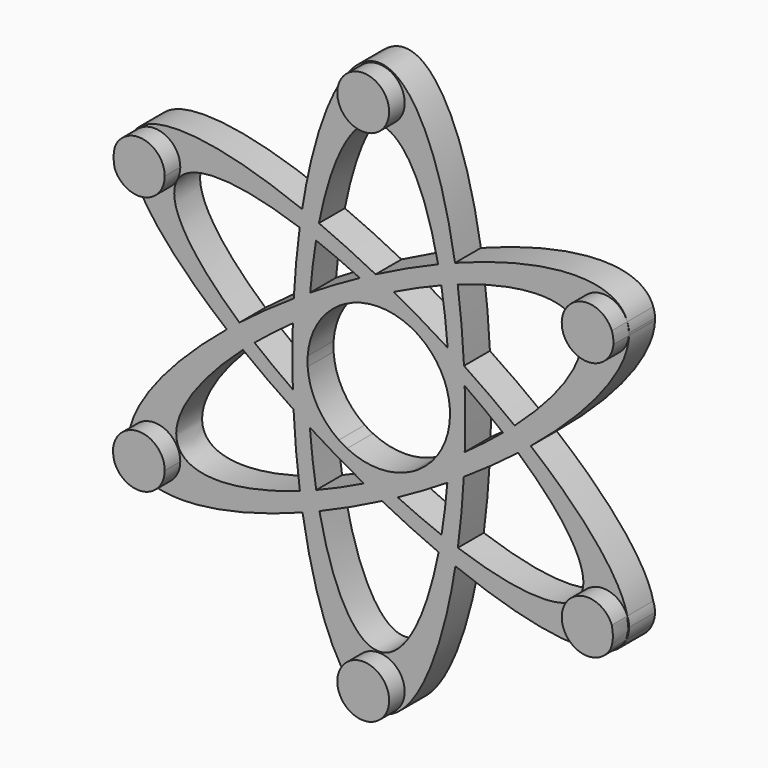
from build123d import *

# Parameters (mm, degrees)
F0_R     = 4
F1_DEPTH = 8
F2_DEPTH = 5


with BuildPart() as f1:
    # F0 (on Front) → F1 (new body)
    with BuildSketch(Plane.XZ):
        with Locations((0, 40)):
            Circle(F0_R)
    extrude(amount=F1_DEPTH)


with BuildPart() as f1b:
    # F0 (on Front) → F1, piece 2 (new body)
    with BuildSketch(Plane.XZ):
        with Locations((0, -40)):
            Circle(F0_R)
    extrude(amount=F1_DEPTH)


with BuildPart() as f1c:
    # F0 (on Front) → F1, piece 3 (new body)
    with BuildSketch(Plane.XZ):
        with BuildLine():
            add(Edge.make_bspline(
                [(38.6271723405, 19.6674961115), (38.6460169038, 20.6376327061), (38.3690323303, 21.4497914918)],
                knots=[2.9551502566, 2.9551502566, 2.9551502566, 3.0789616265, 3.0789616265, 3.0789616265], degree=2, weights=[1, 0.998084455, 1]))
            ThreePointArc((38.3690323303, 21.4497914918), (30.6823221702, 19.4266397613), (38.6271723405, 19.6674961115))
        make_face()
    extrude(amount=F1_DEPTH)


with BuildPart() as f1d:
    # F0 (on Front) → F1, piece 4 (new body)
    with BuildSketch(Plane.XZ):
        with BuildLine():
            add(Edge.make_bspline(
                [(38.1831586596, -21.8582858906), (38.7767020629, -20.4672732588), (38.3678501734, -18.5471723529)],
                knots=[3.1799341158, 3.1799341158, 3.1799341158, 3.4078051361, 3.4078051361, 3.4078051361], degree=2, weights=[1, 0.9935163681, 1]))
            ThreePointArc((38.3678501734, -18.5471723529), (30.6472243235, -19.7772291859), (38.1831586596, -21.8582858906))
        make_face()
    extrude(amount=F1_DEPTH)


with BuildPart() as f1e:
    # F0 (on Front) → F1, piece 5 (new body)
    with BuildSketch(Plane.XZ):
        with BuildLine():
            ThreePointArc((-30.6410161514, 20), (-33.684086173, 23.8838492526), (-38.1831586596, 21.8582858906))
            add(Edge.make_bspline(
                [(-38.1831586596, 21.8582858906), (-38.7767020629, 20.4672732588), (-38.3678501734, 18.5471723529)],
                knots=[0.0383414622, 0.0383414622, 0.0383414622, 0.2662124825, 0.2662124825, 0.2662124825], degree=2, weights=[1, 0.9935163681, 1]))
            ThreePointArc((-38.3678501734, 18.5471723529), (-33.9018734345, 16.068884631), (-30.6410161514, 20))
        make_face()
    extrude(amount=F1_DEPTH)


with BuildPart() as f1f:
    # F0 (on Front) → F1, piece 6 (new body)
    with BuildSketch(Plane.XZ):
        with BuildLine():
            ThreePointArc((-30.6410161514, -20), (-34.4746201727, -16.0034624513), (-38.6271723405, -19.6674961115))
            add(Edge.make_bspline(
                [(-38.6271723405, -19.6674961115), (-38.6460169038, -20.6376327061), (-38.3690323303, -21.4497914918)],
                knots=[6.0967429102, 6.0967429102, 6.0967429102, 6.2205542801, 6.2205542801, 6.2205542801], degree=2, weights=[1, 0.998084455, 1]))
            ThreePointArc((-38.3690323303, -21.4497914918), (-33.9034745307, -23.9314160754), (-30.6410161514, -20))
        make_face()
    extrude(amount=F1_DEPTH)


with BuildPart() as f2:
    # F0 (on Front) → F2 (new body)
    with BuildSketch(Plane.XZ):
        with BuildLine():
            ThreePointArc((38.6271723405, 19.6674961115), (38.6375537001, 19.8336040213), (38.6410161514, 20))
            ThreePointArc((38.6410161514, 20), (38.5724322268, 20.7375416206), (38.3690323303, 21.4497914918))
            add(Edge.make_bspline(
                [(38.6271723405, 19.6674961115), (38.6460169038, 20.6376327061), (38.3690323303, 21.4497914918)],
                knots=[2.9551502566, 2.9551502566, 2.9551502566, 3.0789616265, 3.0789616265, 3.0789616265], degree=2, weights=[1, 0.998084455, 1]))
        make_face()
        with BuildLine():
            add(Edge.make_bspline(
                [(38.6271723405, 19.6674961115), (38.6460169038, 20.6376327061), (38.3690323303, 21.4497914918)],
                knots=[2.9551502566, 2.9551502566, 2.9551502566, 3.0789616265, 3.0789616265, 3.0789616265], degree=2, weights=[1, 0.998084455, 1]))
            ThreePointArc((38.3690323303, 21.4497914918), (30.6823221702, 19.4266397613), (38.6271723405, 19.6674961115))
        make_face()
        with BuildLine():
            ThreePointArc((38.6271723405, 19.6674961115), (30.6823221702, 19.4266397613), (38.3690323303, 21.4497914918))
            add(Edge.make_bspline(
                [(38.3690323303, 21.4497914918), (35.4881888834, 29.8968406764), (11.768870068, 20.7886243591)],
                knots=[3.0789616265, 3.0789616265, 3.0789616265, 4.224226026, 4.224226026, 4.224226026], degree=2, weights=[1, 0.8404776409, 1]))
            add(Edge.make_bspline(
                [(11.768870068, 20.7886243591), (-0.1383581355, 94.7656935014), (-11.8290209253, 20.4105265383)],
                knots=[5.2022540895, 5.2022540895, 5.2022540895, 7.3737896961, 7.3737896961, 7.3737896961], degree=2, weights=[1, 0.4662335933, 1]))
            add(Edge.make_bspline(
                [(-11.8290209253, 20.4105265383), (-34.91761313, 29.5113320816), (-38.1831586596, 21.8582858906)],
                knots=[5.1977622276, 5.1977622276, 5.1977622276, 6.3215267693, 6.3215267693, 6.3215267693], degree=2, weights=[1, 0.8462537744, 1]))
            ThreePointArc((-38.1831586596, 21.8582858906), (-33.684086173, 23.8838492526), (-30.6410161514, 20))
            ThreePointArc((-30.6410161514, 20), (-33.9018734345, 16.068884631), (-38.3678501734, 18.5471723529))
            add(Edge.make_bspline(
                [(-38.3678501734, 18.5471723529), (-36.8074034343, 11.2188090154), (-23.4546094015, 0.2961662725)],
                knots=[0.2662124825, 0.2662124825, 0.2662124825, 1.0897639985, 1.0897639985, 1.0897639985], degree=2, weights=[1, 0.9164115435, 1]))
            add(Edge.make_bspline(
                [(-23.4546094015, 0.2961662725), (-38.4783576877, -12.0063718778), (-38.6271723405, -19.6674961115)],
                knots=[5.1863313593, 5.1863313593, 5.1863313593, 6.0967429102, 6.0967429102, 6.0967429102], degree=2, weights=[1, 0.8981705786, 1]))
            ThreePointArc((-38.6271723405, -19.6674961115), (-34.4746201727, -16.0034624513), (-30.6410161514, -20))
            ThreePointArc((-30.6410161514, -20), (-33.9034745307, -23.9314160754), (-38.3690323303, -21.4497914918))
            add(Edge.make_bspline(
                [(-38.3690323303, -21.4497914918), (-35.4881888834, -29.8968406764), (-11.768870068, -20.7886243591)],
                knots=[6.2205542801, 6.2205542801, 6.2205542801, 7.3658186796, 7.3658186796, 7.3658186796], degree=2, weights=[1, 0.8404776409, 1]))
            add(Edge.make_bspline(
                [(-11.768870068, -20.7886243591), (0.1383581355, -94.7656935014), (11.8290209253, -20.4105265383)],
                knots=[2.060661436, 2.060661436, 2.060661436, 4.2321970425, 4.2321970425, 4.2321970425], degree=2, weights=[1, 0.4662335933, 1]))
            add(Edge.make_bspline(
                [(11.8290209253, -20.4105265383), (34.91761313, -29.5113320816), (38.1831586596, -21.8582858906)],
                knots=[2.056169574, 2.056169574, 2.056169574, 3.1799341158, 3.1799341158, 3.1799341158], degree=2, weights=[1, 0.8462537744, 1]))
            ThreePointArc((38.1831586596, -21.8582858906), (30.6472243235, -19.7772291859), (38.3678501734, -18.5471723529))
            add(Edge.make_bspline(
                [(38.3678501734, -18.5471723529), (36.8074034343, -11.2188090154), (23.4546094015, -0.2961662725)],
                knots=[3.4078051361, 3.4078051361, 3.4078051361, 4.231356652, 4.231356652, 4.231356652], degree=2, weights=[1, 0.9164115435, 1]))
            add(Edge.make_bspline(
                [(23.4546094015, -0.2961662725), (38.4783576877, 12.0063718778), (38.6271723405, 19.6674961115)],
                knots=[2.0447387057, 2.0447387057, 2.0447387057, 2.9551502566, 2.9551502566, 2.9551502566], degree=2, weights=[1, 0.8981705786, 1]))
        make_face()
        with BuildLine():
            add(Edge.make_bspline(
                [(-20.9775166101, -1.6715988722), (-57.3346911932, -34.0027613149), (-12.1812992651, -17.9934813476)],
                knots=[5.2662721481, 5.2662721481, 5.2662721481, 7.272346213, 7.272346213, 7.272346213], degree=2, weights=[1, 0.5377442434, 1]))
            add(Edge.make_bspline(
                [(-20.9775166101, -1.6715988722), (-17.2892670675, -4.5190906219), (-13.156595617, -7.250418808)],
                knots=[1.1684900965, 1.1684900965, 1.1684900965, 1.3957166856, 1.3957166856, 1.3957166856], degree=2, weights=[1, 0.993552949, 1]))
            add(Edge.make_bspline(
                [(-13.156595617, -7.250418808), (-12.8764761834, -12.8287089611), (-12.1812992651, -17.9934813476)],
                knots=[1.73563988, 1.73563988, 1.73563988, 1.9902315228, 1.9902315228, 1.9902315228], degree=2, weights=[1, 0.9919088217, 1]))
        make_face(mode=Mode.SUBTRACT)
        with BuildLine():
            add(Edge.make_bspline(
                [(-10.6355871975, -8.8788558816), (-10.3001887138, -13.1602609633), (-9.6562230523, -17.0474184543)],
                knots=[1.8211625389, 1.8211625389, 1.8211625389, 2.0665528838, 2.0665528838, 2.0665528838], degree=2, weights=[1, 0.9924823853, 1]))
            add(Edge.make_bspline(
                [(-10.6355871975, -8.8788558816), (-6.5457802924, -11.4608048965), (-2.2982627366, -13.7666231954)],
                knots=[1.4645175631, 1.4645175631, 1.4645175631, 1.6844760114, 1.6844760114, 1.6844760114], degree=2, weights=[1, 0.9939583785, 1]))
            add(Edge.make_bspline(
                [(-9.6562230523, -17.0474184543), (-6.06442069, -15.6317314707), (-2.2982627366, -13.7666231954)],
                knots=[1.0753748884, 1.0753748884, 1.0753748884, 1.3157471354, 1.3157471354, 1.3157471354], degree=2, weights=[1, 0.9927863374, 1]))
        make_face(mode=Mode.SUBTRACT)
        with BuildLine():
            add(Edge.make_bspline(
                [(-13.2699308243, 4.4384553681), (-16.4241224972, 2.1873919184), (-19.1756694614, -0.1172964225)],
                knots=[4.9691723309, 4.9691723309, 4.9691723309, 5.191056423, 5.191056423, 5.191056423], degree=2, weights=[1, 0.9938522407, 1]))
            add(Edge.make_bspline(
                [(-13.2699308243, 4.4384553681), (-13.4070301609, -0.0598567192), (-13.2662713173, -4.5569282873)],
                knots=[1.4701714839, 1.4701714839, 1.4701714839, 1.674116558, 1.674116558, 1.674116558], degree=2, weights=[1, 0.9948053046, 1]))
            add(Edge.make_bspline(
                [(-19.1756694614, -0.1172964225), (-16.4170834766, -2.3653682673), (-13.2662713173, -4.5569282873)],
                knots=[1.094094817, 1.094094817, 1.094094817, 1.3131248908, 1.3131248908, 1.3131248908], degree=2, weights=[1, 0.9940092195, 1]))
        make_face(mode=Mode.SUBTRACT)
        with Locations((0, -40)):
            Circle(F0_R, mode=Mode.SUBTRACT)
        with BuildLine():
            add(Edge.make_bspline(
                [(-9.1608560146, -19.7471255553), (-4.4037766582, -17.7758354546), (0.4925988488, -15.2422767275)],
                knots=[1.1527895646, 1.1527895646, 1.1527895646, 1.40497696, 1.40497696, 1.40497696], degree=2, weights=[1, 0.9920607174, 1]))
            add(Edge.make_bspline(
                [(0.4925988488, -15.2422767275), (4.9307327719, -17.5263667759), (9.2397434736, -19.3514863138)],
                knots=[1.7569380094, 1.7569380094, 1.7569380094, 1.9862959493, 1.9862959493, 1.9862959493], degree=2, weights=[1, 0.9934315703, 1]))
            add(Edge.make_bspline(
                [(-9.1608560146, -19.7471255553), (0.1325416539, -65.6909824303), (9.2397434736, -19.3514863138)],
                knots=[2.1543953797, 2.1543953797, 2.1543953797, 4.1419628072, 4.1419628072, 4.1419628072], degree=2, weights=[1, 0.5455226575, 1]))
        make_face(mode=Mode.SUBTRACT)
        with BuildLine():
            add(Edge.make_bspline(
                [(2.9247407794, -13.9530221579), (6.381572516, -15.5960962195), (9.6859688453, -16.866629301)],
                knots=[1.8394563331, 1.8394563331, 1.8394563331, 2.0584655411, 2.0584655411, 2.0584655411], degree=2, weights=[1, 0.9940103597, 1]))
            add(Edge.make_bspline(
                [(2.9247407794, -13.9530221579), (6.8250937635, -11.8359876839), (10.5868988303, -9.4786852371)],
                knots=[1.4680117284, 1.4680117284, 1.4680117284, 1.6698474867, 1.6698474867, 1.6698474867], degree=2, weights=[1, 0.9949121111, 1]))
            add(Edge.make_bspline(
                [(9.6859688453, -16.866629301), (10.2627564961, -13.3368180686), (10.5868988303, -9.4786852371)],
                knots=[4.2223588686, 4.2223588686, 4.2223588686, 4.4447070614, 4.4447070614, 4.4447070614], degree=2, weights=[1, 0.9938265226, 1]))
        make_face(mode=Mode.SUBTRACT)
        with BuildLine():
            add(Edge.make_bspline(
                [(12.2086468073, -17.7889135993), (12.8445989111, -12.9990853571), (13.1252234213, -7.8496558732)],
                knots=[4.2980174693, 4.2980174693, 4.2980174693, 4.533780381, 4.533780381, 4.533780381], degree=2, weights=[1, 0.9930600233, 1]))
            add(Edge.make_bspline(
                [(13.1252234213, -7.8496558732), (17.5751199012, -4.9249756496), (21.5054671299, -1.8547051014)],
                knots=[1.7389094291, 1.7389094291, 1.7389094291, 1.9826652124, 1.9826652124, 1.9826652124], degree=2, weights=[1, 0.9925820789, 1]))
            add(Edge.make_bspline(
                [(12.2086468073, -17.7889135993), (57.3364841528, -33.4072559177), (21.5054671299, -1.8547051014)],
                knots=[2.1436727474, 2.1436727474, 2.1436727474, 4.139111996, 4.139111996, 4.139111996], degree=2, weights=[1, 0.5422197693, 1]))
        make_face(mode=Mode.SUBTRACT)
        with BuildLine():
            add(Edge.make_bspline(
                [(-12.2086468073, 17.7889135993), (-12.8445989111, 12.9990853571), (-13.1252234213, 7.8496558732)],
                knots=[1.1564248157, 1.1564248157, 1.1564248157, 1.3921877274, 1.3921877274, 1.3921877274], degree=2, weights=[1, 0.9930600233, 1]))
            add(Edge.make_bspline(
                [(-13.1252234213, 7.8496558732), (-17.5751199012, 4.9249756496), (-21.5054671299, 1.8547051014)],
                knots=[4.8805020827, 4.8805020827, 4.8805020827, 5.1242578659, 5.1242578659, 5.1242578659], degree=2, weights=[1, 0.9925820789, 1]))
            add(Edge.make_bspline(
                [(-12.2086468073, 17.7889135993), (-57.3364841528, 33.4072559177), (-21.5054671299, 1.8547051014)],
                knots=[5.2852654009, 5.2852654009, 5.2852654009, 7.2807046496, 7.2807046496, 7.2807046496], degree=2, weights=[1, 0.5422197693, 1]))
        make_face(mode=Mode.SUBTRACT)
        with BuildLine():
            add(Edge.make_bspline(
                [(-2.9247407794, 13.9530221579), (-6.381572516, 15.5960962195), (-9.6859688453, 16.866629301)],
                knots=[4.9810489867, 4.9810489867, 4.9810489867, 5.2000581947, 5.2000581947, 5.2000581947], degree=2, weights=[1, 0.9940103597, 1]))
            add(Edge.make_bspline(
                [(-2.9247407794, 13.9530221579), (-6.8250937635, 11.8359876839), (-10.5868988303, 9.4786852371)],
                knots=[4.6096043819, 4.6096043819, 4.6096043819, 4.8114401403, 4.8114401403, 4.8114401403], degree=2, weights=[1, 0.9949121111, 1]))
            add(Edge.make_bspline(
                [(-9.6859688453, 16.866629301), (-10.2627564961, 13.3368180686), (-10.5868988303, 9.4786852371)],
                knots=[1.080766215, 1.080766215, 1.080766215, 1.3031144078, 1.3031144078, 1.3031144078], degree=2, weights=[1, 0.9938265226, 1]))
        make_face(mode=Mode.SUBTRACT)
        with BuildLine():
            add(Edge.make_bspline(
                [(9.1608560146, 19.7471255553), (4.4037766582, 17.7758354546), (-0.4925988488, 15.2422767275)],
                knots=[4.2943822182, 4.2943822182, 4.2943822182, 4.5465696136, 4.5465696136, 4.5465696136], degree=2, weights=[1, 0.9920607174, 1]))
            add(Edge.make_bspline(
                [(-0.4925988488, 15.2422767275), (-4.9307327719, 17.5263667759), (-9.2397434736, 19.3514863138)],
                knots=[4.898530663, 4.898530663, 4.898530663, 5.1278886029, 5.1278886029, 5.1278886029], degree=2, weights=[1, 0.9934315703, 1]))
            add(Edge.make_bspline(
                [(9.1608560146, 19.7471255553), (-0.1325416539, 65.6909824303), (-9.2397434736, 19.3514863138)],
                knots=[5.2959880333, 5.2959880333, 5.2959880333, 7.2835554608, 7.2835554608, 7.2835554608], degree=2, weights=[1, 0.5455226575, 1]))
        make_face(mode=Mode.SUBTRACT)
        with BuildLine():
            ThreePointArc((10.9755620079, 0.7328291827), (10.9938888044, 0.366618271), (11, 0))
            ThreePointArc((11, 0), (10.9938888044, -0.366618271), (10.9755620079, -0.7328291827))
            ThreePointArc((10.9755620079, -0.7328291827), (9.5348282556, -5.4851663728), (6.1508474506, -9.1195984363))
            ThreePointArc((6.1508474506, -9.1195984363), (5.6512634903, -9.4373312416), (5.1353077604, -9.7277239993))
            ThreePointArc((5.1353077604, -9.7277239993), (0.1365678891, -10.9991522042), (-4.8921987801, -9.8522277225))
            ThreePointArc((-4.8921987801, -9.8522277225), (-5.5371729973, -9.5047206797), (-6.1575844575, -9.1150509405))
            ThreePointArc((-6.1575844575, -9.1150509405), (-9.5368541643, -5.4816432435), (-10.9755620079, -0.7328291827))
            ThreePointArc((-10.9755620079, -0.7328291827), (-11, 0), (-10.9755620079, 0.7328291827))
            ThreePointArc((-10.9755620079, 0.7328291827), (-9.5348282556, 5.4851663728), (-6.1508474506, 9.1195984363))
            ThreePointArc((-6.1508474506, 9.1195984363), (-5.6512634903, 9.4373312416), (-5.1353077604, 9.7277239993))
            ThreePointArc((-5.1353077604, 9.7277239993), (-0.1365678891, 10.9991522042), (4.8921987801, 9.8522277225))
            ThreePointArc((4.8921987801, 9.8522277225), (5.5371729973, 9.5047206797), (6.1575844575, 9.1150509405))
            ThreePointArc((6.1575844575, 9.1150509405), (9.5368541643, 5.4816432435), (10.9755620079, 0.7328291827))
        make_face(mode=Mode.SUBTRACT)
        with BuildLine():
            add(Edge.make_bspline(
                [(13.2699308243, -4.4384553681), (16.4241224972, -2.1873919184), (19.1756694614, 0.1172964225)],
                knots=[1.8275796773, 1.8275796773, 1.8275796773, 2.0494637694, 2.0494637694, 2.0494637694], degree=2, weights=[1, 0.9938522407, 1]))
            add(Edge.make_bspline(
                [(13.2699308243, -4.4384553681), (13.4070301609, 0.0598567192), (13.2662713173, 4.5569282873)],
                knots=[4.6117641375, 4.6117641375, 4.6117641375, 4.8157092116, 4.8157092116, 4.8157092116], degree=2, weights=[1, 0.9948053046, 1]))
            add(Edge.make_bspline(
                [(19.1756694614, 0.1172964225), (16.4170834766, 2.3653682673), (13.2662713173, 4.5569282873)],
                knots=[4.2356874706, 4.2356874706, 4.2356874706, 4.4547175444, 4.4547175444, 4.4547175444], degree=2, weights=[1, 0.9940092195, 1]))
        make_face(mode=Mode.SUBTRACT)
        with BuildLine():
            add(Edge.make_bspline(
                [(10.6355871975, 8.8788558816), (10.3001887138, 13.1602609633), (9.6562230523, 17.0474184543)],
                knots=[4.9627551925, 4.9627551925, 4.9627551925, 5.2081455374, 5.2081455374, 5.2081455374], degree=2, weights=[1, 0.9924823853, 1]))
            add(Edge.make_bspline(
                [(10.6355871975, 8.8788558816), (6.5457802924, 11.4608048965), (2.2982627366, 13.7666231954)],
                knots=[4.6061102167, 4.6061102167, 4.6061102167, 4.826068665, 4.826068665, 4.826068665], degree=2, weights=[1, 0.9939583785, 1]))
            add(Edge.make_bspline(
                [(9.6562230523, 17.0474184543), (6.06442069, 15.6317314707), (2.2982627366, 13.7666231954)],
                knots=[4.216967542, 4.216967542, 4.216967542, 4.457339789, 4.457339789, 4.457339789], degree=2, weights=[1, 0.9927863374, 1]))
        make_face(mode=Mode.SUBTRACT)
        with BuildLine():
            add(Edge.make_bspline(
                [(20.9775166101, 1.6715988722), (17.2892670675, 4.5190906219), (13.156595617, 7.250418808)],
                knots=[4.3100827501, 4.3100827501, 4.3100827501, 4.5373093392, 4.5373093392, 4.5373093392], degree=2, weights=[1, 0.993552949, 1]))
            add(Edge.make_bspline(
                [(13.156595617, 7.250418808), (12.8764761834, 12.8287089611), (12.1812992651, 17.9934813476)],
                knots=[4.8772325336, 4.8772325336, 4.8772325336, 5.1318241764, 5.1318241764, 5.1318241764], degree=2, weights=[1, 0.9919088217, 1]))
            add(Edge.make_bspline(
                [(20.9775166101, 1.6715988722), (57.3346911932, 34.0027613149), (12.1812992651, 17.9934813476)],
                knots=[2.1246794946, 2.1246794946, 2.1246794946, 4.1307535594, 4.1307535594, 4.1307535594], degree=2, weights=[1, 0.5377442434, 1]))
        make_face(mode=Mode.SUBTRACT)
        with Locations((0, 40)):
            Circle(F0_R, mode=Mode.SUBTRACT)
        with BuildLine():
            add(Edge.make_bspline(
                [(38.1831586596, -21.8582858906), (38.7767020629, -20.4672732588), (38.3678501734, -18.5471723529)],
                knots=[3.1799341158, 3.1799341158, 3.1799341158, 3.4078051361, 3.4078051361, 3.4078051361], degree=2, weights=[1, 0.9935163681, 1]))
            ThreePointArc((38.3678501734, -18.5471723529), (30.6472243235, -19.7772291859), (38.1831586596, -21.8582858906))
        make_face()
        with BuildLine():
            ThreePointArc((38.6410161514, -20), (38.5721315203, -19.2608572831), (38.3678501734, -18.5471723529))
            add(Edge.make_bspline(
                [(38.1831586596, -21.8582858906), (38.7767020629, -20.4672732588), (38.3678501734, -18.5471723529)],
                knots=[3.1799341158, 3.1799341158, 3.1799341158, 3.4078051361, 3.4078051361, 3.4078051361], degree=2, weights=[1, 0.9935163681, 1]))
            ThreePointArc((38.1831586596, -21.8582858906), (38.5248654039, -20.9569299783), (38.6410161514, -20))
        make_face()
        with BuildLine():
            add(Edge.make_bspline(
                [(-38.1831586596, 21.8582858906), (-38.7767020629, 20.4672732588), (-38.3678501734, 18.5471723529)],
                knots=[0.0383414622, 0.0383414622, 0.0383414622, 0.2662124825, 0.2662124825, 0.2662124825], degree=2, weights=[1, 0.9935163681, 1]))
            ThreePointArc((-38.1831586596, 21.8582858906), (-38.6348079793, 20.2227708141), (-38.3678501734, 18.5471723529))
        make_face()
        with BuildLine():
            ThreePointArc((-30.6410161514, 20), (-33.684086173, 23.8838492526), (-38.1831586596, 21.8582858906))
            add(Edge.make_bspline(
                [(-38.1831586596, 21.8582858906), (-38.7767020629, 20.4672732588), (-38.3678501734, 18.5471723529)],
                knots=[0.0383414622, 0.0383414622, 0.0383414622, 0.2662124825, 0.2662124825, 0.2662124825], degree=2, weights=[1, 0.9935163681, 1]))
            ThreePointArc((-38.3678501734, 18.5471723529), (-33.9018734345, 16.068884631), (-30.6410161514, 20))
        make_face()
        with BuildLine():
            add(Edge.make_bspline(
                [(-38.6271723405, -19.6674961115), (-38.6460169038, -20.6376327061), (-38.3690323303, -21.4497914918)],
                knots=[6.0967429102, 6.0967429102, 6.0967429102, 6.2205542801, 6.2205542801, 6.2205542801], degree=2, weights=[1, 0.998084455, 1]))
            ThreePointArc((-38.6271723405, -19.6674961115), (-38.5997101326, -20.5733602387), (-38.3690323303, -21.4497914918))
        make_face()
        with BuildLine():
            ThreePointArc((-30.6410161514, -20), (-34.4746201727, -16.0034624513), (-38.6271723405, -19.6674961115))
            add(Edge.make_bspline(
                [(-38.6271723405, -19.6674961115), (-38.6460169038, -20.6376327061), (-38.3690323303, -21.4497914918)],
                knots=[6.0967429102, 6.0967429102, 6.0967429102, 6.2205542801, 6.2205542801, 6.2205542801], degree=2, weights=[1, 0.998084455, 1]))
            ThreePointArc((-38.3690323303, -21.4497914918), (-33.9034745307, -23.9314160754), (-30.6410161514, -20))
        make_face()
    extrude(amount=F2_DEPTH)


solid = Compound([f1.part, f1b.part, f1c.part, f1d.part, f1e.part, f1f.part, f2.part])
